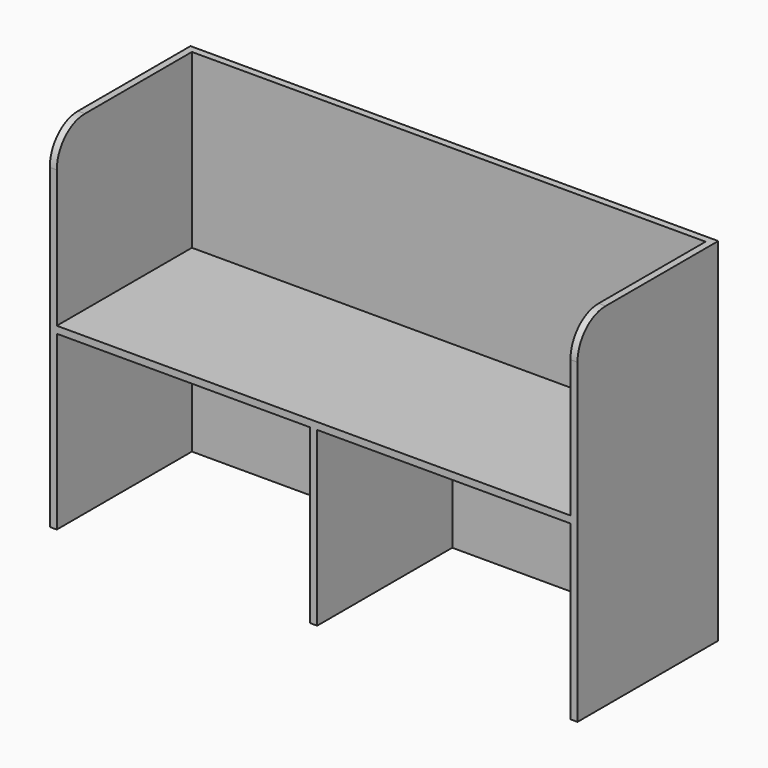
from build123d import *

# Parameters (mm, degrees)
F0_W     = 750
F0_H     = 250
F1_DEPTH = 250
F3_T     = -10
F4_W     = 730
F4_H     = 240
F5_DEPTH = 5
F6_R     = 50
F8_W     = 240
F8_H     = 245
F9_DEPTH = 5


# Not quite as in the source:
# - a feature of the source that left no trace in its solid (it failed there, or was rolled back) is left out


with BuildPart() as f1:
    # F0 (on Front) → F1 (new body)
    with BuildSketch(Plane.XZ):
        with Locations((0, 125)):
            Rectangle(F0_W, F0_H)
    extrude(amount=-F1_DEPTH)

    # F2: F1 across plane


with BuildPart() as f1_1:
    add(f1.part)
    add(f1.part.mirror(Plane.XY))

    # F3
    f3_openings = [f1_1.faces().sort_by_distance(p)[0] for p in [
        (0, 0, 0),
        (0, 125, 250),
        (0, 125, -250),
    ]]
    offset(amount=F3_T, openings=f3_openings)

    # F4 (on Top) → F5 (join, symmetric)
    with BuildSketch(Plane.XY):
        with Locations((0, 120)):
            Rectangle(F4_W, F4_H)
    extrude(amount=F5_DEPTH, both=True)

    # F6
    f6_edges = [f1_1.edges().sort_by_distance(p)[0] for p in [
        (-370, 0, 250),
        (370, 0, 250),
    ]]
    fillet(f6_edges, radius=F6_R)

    # F8 (on Right) → F9 (join, symmetric)
    with BuildSketch(Plane.YZ):
        with Locations((120, -127.5)):
            Rectangle(F8_W, F8_H)
    extrude(amount=F9_DEPTH, both=True)


solid = f1_1.part
